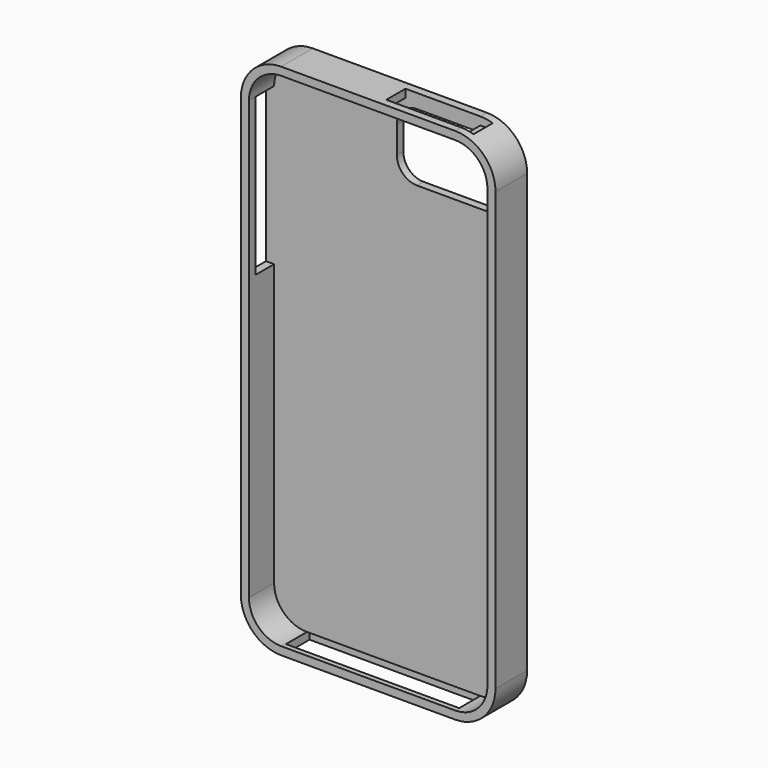
from build123d import *

# Parameters (mm, degrees)
F1_DEPTH  = 7.8
F2_T      = 2
F4_DEPTH  = 9.801
F5_W      = 45.0870413333
F5_H      = 7.3114127154
F6_DEPTH  = 2
F7_W      = 5.831967108
F7_H      = 39.9042963982
F8_DEPTH  = 2
F9_W      = 21.6295962455
F9_H      = 5.9405225329
F10_DEPTH = 2
F13_DEPTH = 7
F16_DEPTH = 2
F14_R     = 4.5
F14_R_2   = 6
F17_DEPTH = 155
F18_DEPTH = 5


# Not quite as in the source:
# - an extrude ends at something that could not be found from the text; its depth is read off the source's solid


with BuildPart() as f1:
    # F0 (on Front) → F1 (new body)
    with BuildSketch(Plane.XZ):
        with BuildLine():
            Line((-23.3265317287, -64.975), (19.7734682713, -64.975))
            ThreePointArc((19.7734682713, -64.975), (25.4303225208, -62.6318542495), (27.7734682713, -56.975))
            Line((27.7734682713, -56.975), (27.7734682713, 51.465))
            ThreePointArc((27.7734682713, 51.465), (25.4303225208, 57.1218542495), (19.7734682713, 59.465))
            Line((19.7734682713, 59.465), (-23.3265317287, 59.465))
            ThreePointArc((-23.3265317287, 59.465), (-28.9833859782, 57.1218542495), (-31.3265317287, 51.465))
            Line((-31.3265317287, 51.465), (-31.3265317287, -56.975))
            ThreePointArc((-31.3265317287, -56.975), (-28.9833859782, -62.6318542495), (-23.3265317287, -64.975))
        make_face()
    extrude(amount=F1_DEPTH)

    # F2
    f2_openings = [f1.faces().sort_by_distance(p)[0] for p in [
        (-1.776532, -7.8, -2.755),
    ]]
    offset(amount=F2_T, openings=f2_openings, kind=Kind.INTERSECTION)

    # F3 (on face) → F4 (cut, through all)
    with BuildSketch(Plane(origin=(0, 2, 0), x_dir=(-1, 0, 0), z_dir=(0, 1, 0))):
        with BuildLine():
            Line((-4.0860684775, 57.9532251436), (-20.8159385248, 57.9532251436))
            ThreePointArc((-20.8159385248, 57.9532251436), (-24.3514724307, 56.4887590495), (-25.8159385248, 52.9532251436))
            Line((-25.8159385248, 52.9532251436), (-25.8159385248, 46.2790104747))
            ThreePointArc((-25.8159385248, 46.2790104747), (-24.3514724307, 42.7434765687), (-20.8159385248, 41.2790104747))
            Line((-20.8159385248, 41.2790104747), (-4.0860684775, 41.2790104747))
            ThreePointArc((-4.0860684775, 41.2790104747), (-0.5505345715, 42.7434765687), (0.9139315225, 46.2790104747))
            Line((0.9139315225, 46.2790104747), (0.9139315225, 52.9532251436))
            ThreePointArc((0.9139315225, 52.9532251436), (-0.5505345715, 56.4887590495), (-4.0860684775, 57.9532251436))
        make_face()
    extrude(amount=-F4_DEPTH, mode=Mode.SUBTRACT)

    # F5 (on face) → F6 (cut)
    with BuildSketch(Plane(origin=(0, 0, -66.975), x_dir=(1, 0, 0), z_dir=(0, 0, -1))):
        with Locations((-0.6092851982, 2.8941009077)):
            Rectangle(F5_W, F5_H)
    extrude(amount=-F6_DEPTH, mode=Mode.SUBTRACT)

    # F7 (on face) → F8 (cut)
    with BuildSketch(Plane(origin=(-33.3265317287, 0, 0), x_dir=(0, -1, 0), z_dir=(-1, 0, 0))):
        with Locations((2.915983554, 32.564714551)):
            Rectangle(F7_W, F7_H)
    extrude(amount=-F8_DEPTH, mode=Mode.SUBTRACT)

    # F9 (on face) → F10 (cut)
    with BuildSketch(Plane.XY.offset(61.465)):
        with Locations((12.0333628147, -2.9702612665)):
            Rectangle(F9_W, F9_H)
    extrude(amount=-F10_DEPTH, mode=Mode.SUBTRACT)

    # F14 (on face) → F17 (cut, through all)
    with BuildSketch(Plane(origin=(0, 9, 0), x_dir=(-1, 0, 0), z_dir=(0, 1, 0))):
        with Locations((-7.0430367999, -6.644173318)):
            Circle(F14_R)
        with Locations((7.9569632001, -6.644173318)):
            Circle(F14_R)
        with Locations((-7.0430367999, -21.644173318)):
            Circle(F14_R_2)
        with Locations((7.9569632001, -21.644173318)):
            Circle(F14_R_2)
    extrude(amount=F17_DEPTH, mode=Mode.SUBTRACT)


with BuildPart() as f13:
    # F12 (on face) → F13 (new body)
    with BuildSketch(Plane(origin=(0, 2, 0), x_dir=(-1, 0, 0), z_dir=(0, 1, 0))):
        with BuildLine():
            ThreePointArc((-14.0430367999, -21.644173318), (-11.9927842682, -26.5939207863), (-7.0430367999, -28.644173318))
            Line((-7.0430367999, -28.644173318), (7.9569632001, -28.644173318))
            ThreePointArc((7.9569632001, -28.644173318), (12.9067106684, -26.5939207863), (14.9569632001, -21.644173318))
            Line((14.9569632001, -21.644173318), (14.9569632001, -6.644173318))
            ThreePointArc((14.9569632001, -6.644173318), (12.9067106684, -1.6944258497), (7.9569632001, 0.355826682))
            Line((7.9569632001, 0.355826682), (-7.0430367999, 0.355826682))
            ThreePointArc((-7.0430367999, 0.355826682), (-11.9927842682, -1.6944258497), (-14.0430367999, -6.644173318))
            Line((-14.0430367999, -6.644173318), (-14.0430367999, -21.644173318))
        make_face()
    extrude(amount=F13_DEPTH)

    # F15 (on face) → F16 (join)
    with BuildSketch(Plane(origin=(0, 9, 0), x_dir=(-1, 0, 0), z_dir=(0, 1, 0))):
        with BuildLine():
            Line((7.9569632001, 4.4558267109), (-7.0430367999, 4.4558267109))
            ThreePointArc((-7.0430367999, 4.4558267109), (-14.8919220915, 1.2047119736), (-18.1430368288, -6.644173318))
            Line((-18.1430368288, -6.644173318), (-18.1430368288, -21.644173318))
            ThreePointArc((-18.1430368288, -21.644173318), (-14.8919220915, -29.4930586096), (-7.0430367999, -32.7441733469))
            Line((-7.0430367999, -32.7441733469), (7.9569632001, -32.7441733469))
            ThreePointArc((7.9569632001, -32.7441733469), (15.8058484917, -29.4930586096), (19.056963229, -21.644173318))
            Line((19.056963229, -21.644173318), (19.056963229, -6.644173318))
            ThreePointArc((19.056963229, -6.644173318), (15.8058484917, 1.2047119736), (7.9569632001, 4.4558267109))
        make_face()
        with BuildLine():
            Line((-14.0430367999, -21.644173318), (-14.0430367999, -6.644173318))
            ThreePointArc((-14.0430367999, -6.644173318), (-11.9927842682, -1.6944258497), (-7.0430367999, 0.355826682))
            Line((-7.0430367999, 0.355826682), (7.9569632001, 0.355826682))
            ThreePointArc((7.9569632001, 0.355826682), (12.9067106684, -1.6944258497), (14.9569632001, -6.644173318))
            Line((14.9569632001, -6.644173318), (14.9569632001, -21.644173318))
            ThreePointArc((14.9569632001, -21.644173318), (12.9067106684, -26.5939207863), (7.9569632001, -28.644173318))
            Line((7.9569632001, -28.644173318), (-7.0430367999, -28.644173318))
            ThreePointArc((-7.0430367999, -28.644173318), (-11.9927842682, -26.5939207863), (-14.0430367999, -21.644173318))
        make_face(mode=Mode.SUBTRACT)
    extrude(amount=-F16_DEPTH)

    # F14 (on face) → F18 (cut)
    with BuildSketch(Plane(origin=(0, 9, 0), x_dir=(-1, 0, 0), z_dir=(0, 1, 0))):
        with Locations((7.9569632001, -6.644173318)):
            Circle(F14_R)
        with Locations((-7.0430367999, -6.644173318)):
            Circle(F14_R)
        with Locations((-7.0430367999, -21.644173318)):
            Circle(F14_R_2)
        with Locations((7.9569632001, -21.644173318)):
            Circle(F14_R_2)
    extrude(amount=-F18_DEPTH, mode=Mode.SUBTRACT)


solid = Compound([f1.part, f13.part])
